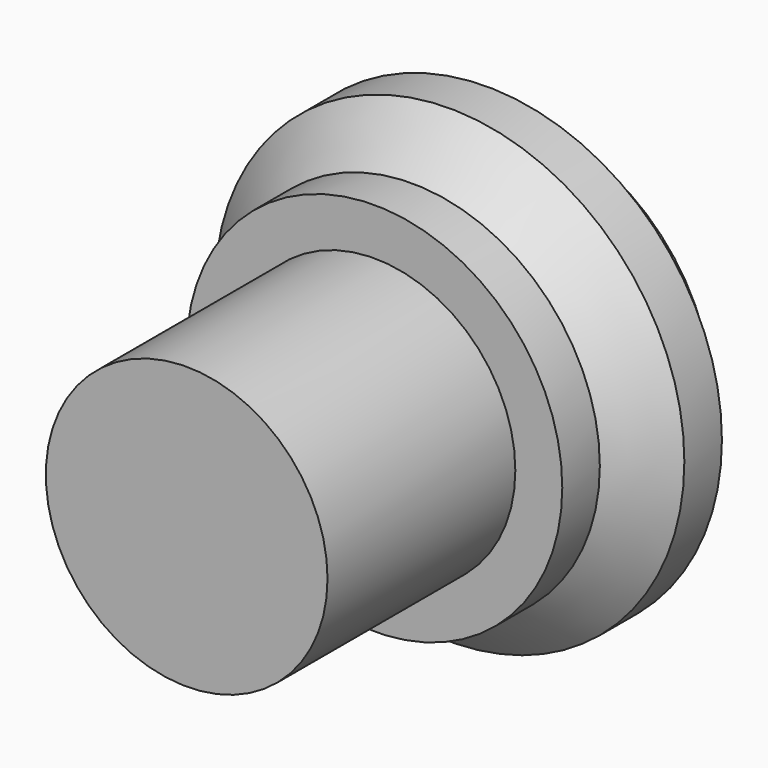
from build123d import *

# Parameters (mm, degrees)
F0_R        = 10
F0_R_2      = 7.5
F1_DEPTH    = 2.5
F1_FACE_R   = 10
F1_FACE_R_2 = 7.5
F2_R        = 12.5
F2_R_2      = 10
F3_DEPTH    = 5
F4_R        = 10
F4_R_2      = 7.5
F5_DEPTH    = 2.5
F7_SIZE     = 2.49999
F8_R        = 5
F6_R        = 7.5
F9_DEPTH    = 20


# Not quite as in the source:
# - a fillet or chamfer is up to 0.001 mm smaller than in the source, because OpenCascade refuses the exact size


with BuildPart() as f1:
    # F0 (on Front) → F1 (new body)
    with BuildSketch(Plane.XZ):
        Circle(F0_R)
        Circle(F0_R_2, mode=Mode.SUBTRACT)
    extrude(amount=F1_DEPTH)

    # F1_face (on face) + F2 (on Front) → F3 (join)
    with BuildSketch(Plane.XZ.offset(2.5)):
        Circle(F1_FACE_R)
        Circle(F1_FACE_R_2, mode=Mode.SUBTRACT)
    with BuildSketch(Plane.XZ):
        Circle(F2_R)
        Circle(F2_R_2, mode=Mode.SUBTRACT)
    extrude(amount=F3_DEPTH)

    # F4 (on Front) → F5 (join)
    with BuildSketch(Plane.XZ):
        Circle(F4_R)
        Circle(F4_R_2, mode=Mode.SUBTRACT)
    extrude(amount=-F5_DEPTH)

    # F7 (size 2.5 in the source; OpenCascade refuses exactly that, so slightly less here)
    f7_edges = [f1.edges().sort_by_distance(p)[0] for p in [
        (-12.5, -5, 0),
    ]]
    chamfer(f7_edges, length=F7_SIZE)

    # F8 (on Front) + F6 (on Front) → F9 (join)
    with BuildSketch(Plane.XZ):
        Circle(F8_R)
    with BuildSketch(Plane.XZ):
        Circle(F6_R)
    extrude(amount=F9_DEPTH)


solid = f1.part
